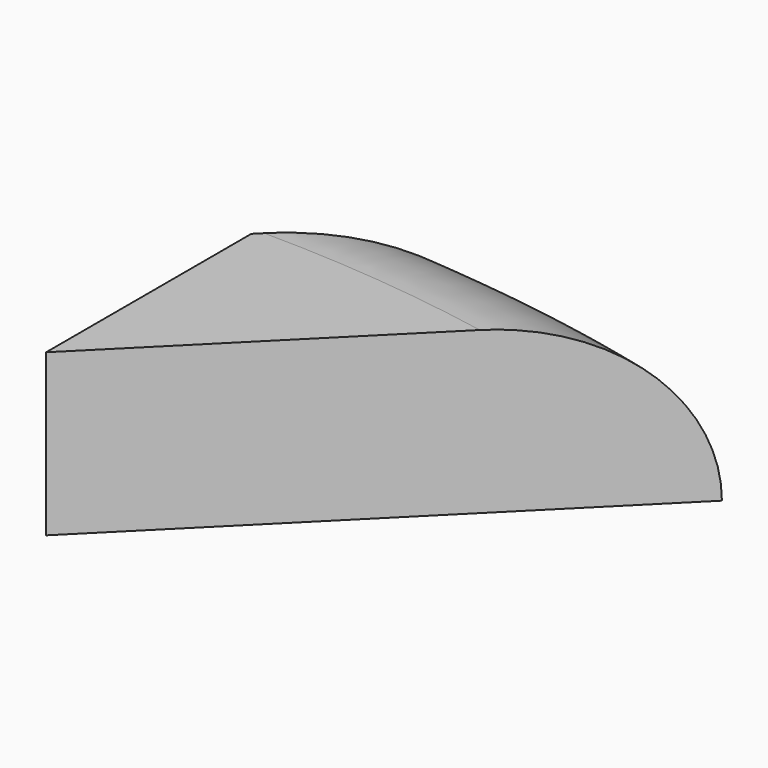
from build123d import *

# Parameters (mm, degrees)
F2_DEPTH = 25.4
F3_R     = 25.39999


# Not quite as in the source:
# - a fillet or chamfer is up to 0.001 mm smaller than in the source, because OpenCascade refuses the exact size


with BuildPart() as f2:
    # F1 (on face) → F2 (new body)
    with BuildSketch(Plane.XY):
        with BuildLine():
            Line((25.1559020156, 227.2116647397), (0, 202.0557627241))
            Line((0, 202.0557627241), (0, 161.6446101792))
            Line((0, 161.6446101792), (59.1660337104, 220.8106438897))
            ThreePointArc((59.1660337104, 220.8106438897), (42.28227144, 224.6556687953), (25.1559020156, 227.2116647397))
        make_face()
    extrude(amount=F2_DEPTH)

    # F3 (radius 25.4 in the source; OpenCascade refuses exactly that, so slightly less here)
    f3_edges = [f2.edges().sort_by_distance(p)[0] for p in [
        (42.282271, 224.655669, 25.4),
    ]]
    fillet(f3_edges, radius=F3_R)


solid = f2.part
